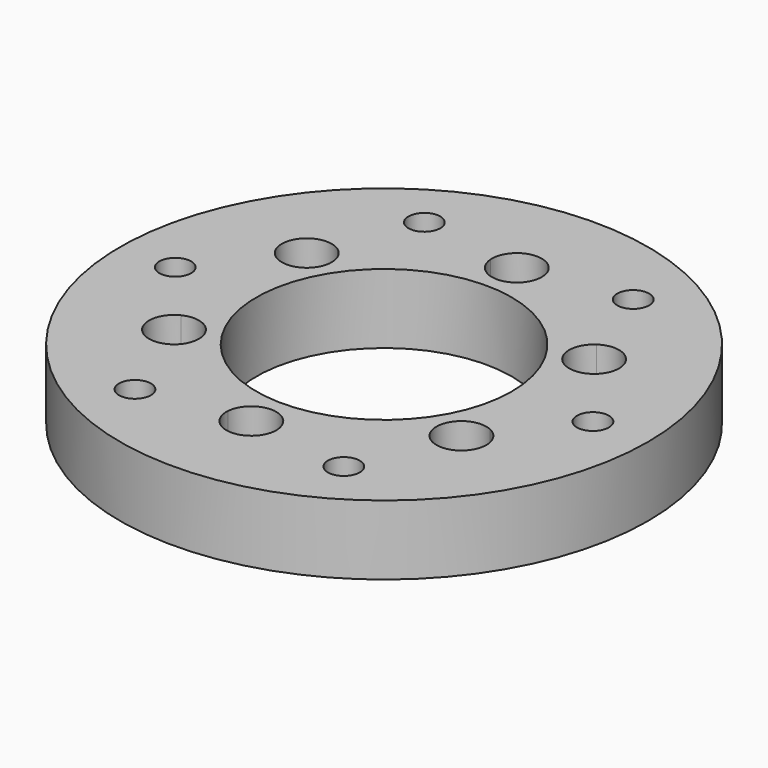
from build123d import *

# Parameters (mm, degrees)
F0_R     = 45.5
F0_R_2   = 2.75
F0_R_3   = 2.05
F0_R_4   = 22
F1_DEPTH = 12
F3_DEPTH = 5.1


# Not quite as in the source:
# - a feature names something its author has since deleted; it is built from what else it names


with BuildPart() as f1:
    # F0 (on Top) → F1 (new body)
    with BuildSketch(Plane.XY):
        Circle(F0_R)
        with Locations((-18, -31.1769145362)):
            Circle(F0_R_2, mode=Mode.SUBTRACT)
        with Locations((-24.7683265482, -14.3)):
            Circle(F0_R_3, mode=Mode.SUBTRACT)
        with Locations((0, -28.6)):
            Circle(F0_R_3, mode=Mode.SUBTRACT)
        with Locations((18, -31.1769145362)):
            Circle(F0_R_2, mode=Mode.SUBTRACT)
        with Locations((24.7683265482, -14.3)):
            Circle(F0_R_3, mode=Mode.SUBTRACT)
        with Locations((-36, 0)):
            Circle(F0_R_2, mode=Mode.SUBTRACT)
        with Locations((-24.7683265482, 14.3)):
            Circle(F0_R_3, mode=Mode.SUBTRACT)
        with Locations((-18, 31.1769145362)):
            Circle(F0_R_2, mode=Mode.SUBTRACT)
        Circle(F0_R_4, mode=Mode.SUBTRACT)
        with Locations((36, 0)):
            Circle(F0_R_2, mode=Mode.SUBTRACT)
        with Locations((24.7683265482, 14.3)):
            Circle(F0_R_3, mode=Mode.SUBTRACT)
        with Locations((0, 28.6)):
            Circle(F0_R_3, mode=Mode.SUBTRACT)
        with Locations((18, 31.1769145362)):
            Circle(F0_R_2, mode=Mode.SUBTRACT)
    extrude(amount=F1_DEPTH)

    # F2 (on face) → F3 (cut)
    with BuildSketch(Plane.XY.offset(12)):
        with BuildLine():
            ThreePointArc((-20.4683265482, 14.3), (-20.9661824008, 16.3084072998), (-22.3444660282, 17.8517460747))
            ThreePointArc((-22.3444660282, 17.8517460747), (-23.0302843715, 16.957771132), (-23.6803579094, 16.0374764001))
            ThreePointArc((-23.6803579094, 16.0374764001), (-22.9748891072, 15.2930166893), (-22.7183265482, 14.3))
            ThreePointArc((-22.7183265482, 14.3), (-23.7116725089, 12.5433036002), (-25.7290409298, 12.4890533202))
            ThreePointArc((-25.7290409298, 12.4890533202), (-26.2010027777, 11.4659257561), (-26.6322986167, 10.425002177))
            ThreePointArc((-26.6322986167, 10.425002177), (-22.4797767776, 10.6595961835), (-20.4683265482, 14.3))
        make_face()
        with BuildLine():
            ThreePointArc((-23.6803579094, 16.0374764001), (-23.0302843715, 16.957771132), (-22.3444660282, 17.8517460747))
            ThreePointArc((-22.3444660282, 17.8517460747), (-28.4922357845, 16.45), (-26.6322986167, 10.425002177))
            ThreePointArc((-26.6322986167, 10.425002177), (-26.2010027777, 11.4659257561), (-25.7290409298, 12.4890533202))
            ThreePointArc((-25.7290409298, 12.4890533202), (-26.543678626, 15.325), (-23.6803579094, 16.0374764001))
        make_face()
        with BuildLine():
            ThreePointArc((2.0486830204, 28.5265297203), (3.1707184061, 28.4236968881), (4.2878325885, 28.2767482517))
            ThreePointArc((4.2878325885, 28.2767482517), (4.2969570705, 28.438259669), (4.3, 28.6))
            ThreePointArc((4.3, 28.6), (-0.161740331, 32.8969570705), (-4.2878325885, 28.2767482517))
            ThreePointArc((-4.2878325885, 28.2767482517), (-3.1707184061, 28.4236968881), (-2.0486830204, 28.5265297203))
            ThreePointArc((-2.0486830204, 28.5265297203), (-0.0367410412, 30.6496707287), (2.05, 28.6))
            ThreePointArc((2.05, 28.6), (2.0496707287, 28.5632589588), (2.0486830204, 28.5265297203))
        make_face()
        with BuildLine():
            ThreePointArc((-4.2878325885, 28.2767482517), (0, 24.3), (4.2878325885, 28.2767482517))
            ThreePointArc((4.2878325885, 28.2767482517), (3.1707184061, 28.4236968881), (2.0486830204, 28.5265297203))
            ThreePointArc((2.0486830204, 28.5265297203), (0, 26.55), (-2.0486830204, 28.5265297203))
            ThreePointArc((-2.0486830204, 28.5265297203), (-3.1707184061, 28.4236968881), (-4.2878325885, 28.2767482517))
        make_face()
        with BuildLine():
            ThreePointArc((25.7290409298, 12.4890533202), (26.2010027777, 11.4659257561), (26.6322986167, 10.425002177))
            ThreePointArc((26.6322986167, 10.425002177), (28.4087303647, 12.0114502293), (29.0683265482, 14.3))
            ThreePointArc((29.0683265482, 14.3), (26.776733848, 18.1021441475), (22.3444660282, 17.8517460747))
            ThreePointArc((22.3444660282, 17.8517460747), (23.0302843715, 16.957771132), (23.6803579094, 16.0374764001))
            ThreePointArc((23.6803579094, 16.0374764001), (25.7613432375, 16.093437441), (26.8183265482, 14.3))
            ThreePointArc((26.8183265482, 14.3), (26.525022948, 13.2433459606), (25.7290409298, 12.4890533202))
        make_face()
        with BuildLine():
            ThreePointArc((22.3444660282, 17.8517460747), (21.044417312, 12.15), (26.6322986167, 10.425002177))
            ThreePointArc((26.6322986167, 10.425002177), (26.2010027777, 11.4659257561), (25.7290409298, 12.4890533202))
            ThreePointArc((25.7290409298, 12.4890533202), (22.9929744705, 13.275), (23.6803579094, 16.0374764001))
            ThreePointArc((23.6803579094, 16.0374764001), (23.0302843715, 16.957771132), (22.3444660282, 17.8517460747))
        make_face()
        with BuildLine():
            ThreePointArc((29.0683265482, -14.3), (28.4087303647, -12.0114502293), (26.6322986167, -10.425002177))
            ThreePointArc((26.6322986167, -10.425002177), (26.2010027777, -11.4659257561), (25.7290409298, -12.4890533202))
            ThreePointArc((25.7290409298, -12.4890533202), (26.525022948, -13.2433459606), (26.8183265482, -14.3))
            ThreePointArc((26.8183265482, -14.3), (25.7613432375, -16.093437441), (23.6803579094, -16.0374764001))
            ThreePointArc((23.6803579094, -16.0374764001), (23.0302843715, -16.957771132), (22.3444660282, -17.8517460747))
            ThreePointArc((22.3444660282, -17.8517460747), (26.776733848, -18.1021441475), (29.0683265482, -14.3))
        make_face()
        with BuildLine():
            ThreePointArc((25.7290409298, -12.4890533202), (26.2010027777, -11.4659257561), (26.6322986167, -10.425002177))
            ThreePointArc((26.6322986167, -10.425002177), (21.044417312, -12.15), (22.3444660282, -17.8517460747))
            ThreePointArc((22.3444660282, -17.8517460747), (23.0302843715, -16.957771132), (23.6803579094, -16.0374764001))
            ThreePointArc((23.6803579094, -16.0374764001), (22.9929744705, -13.275), (25.7290409298, -12.4890533202))
        make_face()
        with BuildLine():
            ThreePointArc((2.0486830204, -28.5265297203), (3.1707184061, -28.4236968881), (4.2878325885, -28.2767482517))
            ThreePointArc((4.2878325885, -28.2767482517), (0, -24.3), (-4.2878325885, -28.2767482517))
            ThreePointArc((-4.2878325885, -28.2767482517), (-3.1707184061, -28.4236968881), (-2.0486830204, -28.5265297203))
            ThreePointArc((-2.0486830204, -28.5265297203), (0, -26.55), (2.0486830204, -28.5265297203))
        make_face()
        with BuildLine():
            ThreePointArc((4.3, -28.6), (4.2969570705, -28.438259669), (4.2878325885, -28.2767482517))
            ThreePointArc((4.2878325885, -28.2767482517), (3.1707184061, -28.4236968881), (2.0486830204, -28.5265297203))
            ThreePointArc((2.0486830204, -28.5265297203), (2.0496707287, -28.5632589588), (2.05, -28.6))
            ThreePointArc((2.05, -28.6), (-0.0367410412, -30.6496707287), (-2.0486830204, -28.5265297203))
            ThreePointArc((-2.0486830204, -28.5265297203), (-3.1707184061, -28.4236968881), (-4.2878325885, -28.2767482517))
            ThreePointArc((-4.2878325885, -28.2767482517), (-0.161740331, -32.8969570705), (4.3, -28.6))
        make_face()
        with BuildLine():
            ThreePointArc((-23.6803579094, -16.0374764001), (-23.0302843715, -16.957771132), (-22.3444660282, -17.8517460747))
            ThreePointArc((-22.3444660282, -17.8517460747), (-20.9661824008, -16.3084072998), (-20.4683265482, -14.3))
            ThreePointArc((-20.4683265482, -14.3), (-22.4797767776, -10.6595961835), (-26.6322986167, -10.425002177))
            ThreePointArc((-26.6322986167, -10.425002177), (-26.2010027777, -11.4659257561), (-25.7290409298, -12.4890533202))
            ThreePointArc((-25.7290409298, -12.4890533202), (-23.7116725089, -12.5433036002), (-22.7183265482, -14.3))
            ThreePointArc((-22.7183265482, -14.3), (-22.9748891072, -15.2930166893), (-23.6803579094, -16.0374764001))
        make_face()
        with BuildLine():
            ThreePointArc((-26.6322986167, -10.425002177), (-28.4922357845, -16.45), (-22.3444660282, -17.8517460747))
            ThreePointArc((-22.3444660282, -17.8517460747), (-23.0302843715, -16.957771132), (-23.6803579094, -16.0374764001))
            ThreePointArc((-23.6803579094, -16.0374764001), (-26.543678626, -15.325), (-25.7290409298, -12.4890533202))
            ThreePointArc((-25.7290409298, -12.4890533202), (-26.2010027777, -11.4659257561), (-26.6322986167, -10.425002177))
        make_face()
    extrude(amount=-F3_DEPTH, mode=Mode.SUBTRACT)


solid = f1.part
